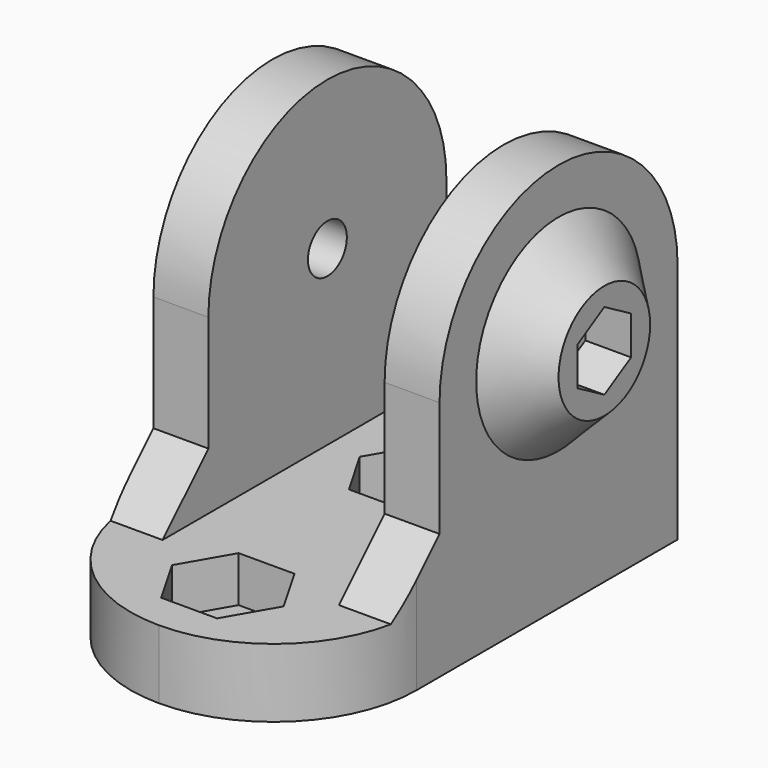
from build123d import *

# Parameters (mm, degrees)
F0_R      = 2.125
F1_DEPTH  = 12.5
F2_W      = 15.4
F2_H      = 26
F3_DEPTH  = 28.101
F4_R      = 2.25
F5_DEPTH  = 25
F7_DEPTH  = 4
F8_R      = 12.49999
F9_SIZE   = 5
F10_R     = 5
F11_DEPTH = 4
F12_SIZE  = 3.99999


# Not quite as in the source:
# - a fillet or chamfer is up to 0.001 mm smaller than in the source, because OpenCascade refuses the exact size
# - a feature names something its author has since deleted; it is built from what else it names


with BuildPart() as f1:
    # F0 (on Right) → F1 (new body, symmetric)
    with BuildSketch(Plane.YZ):
        with BuildLine():
            Line((13, -15.1), (13, 0))
            ThreePointArc((13, 0), (0, 13), (-13, 0))
            Line((-13, 0), (-13, -15.1))
            Line((-13, -15.1), (-28, -15.1))
            Line((-28, -15.1), (-28, -21.1))
            Line((-28, -21.1), (0, -21.1))
            Line((0, -21.1), (13, -21.1))
            Line((13, -21.1), (13, -15.1))
        make_face()
        Circle(F0_R, mode=Mode.SUBTRACT)
    extrude(amount=F1_DEPTH, both=True)

    # F2 (on face) → F3 (cut, through all)
    with BuildSketch(Plane.XY.offset(-15.1)):
        Rectangle(F2_W, F2_H)
    extrude(amount=F3_DEPTH, mode=Mode.SUBTRACT)

    # F4 (on face) → F5 (cut)
    with BuildSketch(Plane.XY.offset(-15.1)):
        with Locations((0, -20.5)):
            Circle(F4_R)
        Circle(F4_R)
    extrude(amount=-F5_DEPTH, mode=Mode.SUBTRACT)

    # F6 (on face) → F7 (cut)
    with BuildSketch(Plane.XY.offset(-15.1)):
        Polygon((-4.8786097747, -20.5), (-2.4393048873, -24.725), (2.4393048873, -24.725), (4.8786097747, -20.5), (2.4393048873, -16.275), (-2.4393048873, -16.275), align=None)
        Polygon((2.4393048873, 4.225), (-2.4393048873, 4.225), (-4.8786097747, 0), (-2.4393048873, -4.225), (2.4393048873, -4.225), (4.8786097747, 0), align=None)
    extrude(amount=-F7_DEPTH, mode=Mode.SUBTRACT)

    # F8 (radius 12.5 in the source; OpenCascade refuses exactly that, so slightly less here)
    f8_edges = [f1.edges().sort_by_distance(p)[0] for p in [
        (-12.5, -28, -18.1),
        (12.5, -28, -18.1),
    ]]
    fillet(f8_edges, radius=F8_R)

    # F9
    f9_edges = [f1.edges().sort_by_distance(p)[0] for p in [
        (-10.1, -13, -15.1),
        (10.1, -13, -15.1),
        (10.1, 13, 0),
        (-10.1, 13, 0),
    ]]
    chamfer(f9_edges, length=F9_SIZE)

    # F10 (on face) → F11 (join)
    with BuildSketch(Plane.YZ.offset(12.5)):
        Circle(F10_R)
        Polygon((0, 3.3746123234), (2.9225, 1.6873061617), (2.9225, -1.6873061617), (0, -3.3746123234), (-2.9225, -1.6873061617), (-2.9225, 1.6873061617), align=None, mode=Mode.SUBTRACT)
    extrude(amount=F11_DEPTH)

    # F12 (size 4 in the source; OpenCascade refuses exactly that, so slightly less here)
    f12_edges = [f1.edges().sort_by_distance(p)[0] for p in [
        (12.5, -5, 0),
    ]]
    chamfer(f12_edges, length=F12_SIZE)


solid = f1.part
